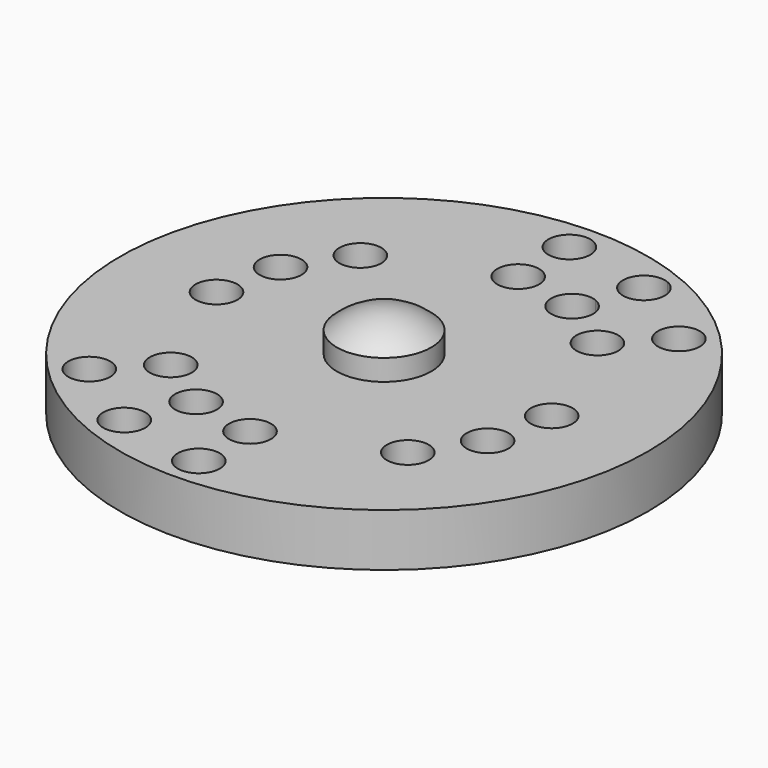
from build123d import *

# Parameters (mm, degrees)
F0_W     = 1.7891867319
F0_H     = 0.8
F2_R     = 0.79375
F3_DEPTH = 25.4


with BuildPart() as f1:
    # F0 (on Front) → F1 (revolve)
    with BuildSketch(Plane.XZ):
        with Locations((0.894593366, 0.4)):
            Rectangle(F0_W, F0_H)
        Polygon((1.7891867319, 0), (0, 0), (0, -3), (2.2, -3), (2.2, -2), (10, -2), (10, 0), align=None)
    revolve(axis=Axis((0, 0, -1.5), (0, 0, 1)))

    # F2 (on face) → F3 (cut)
    with BuildSketch(Plane.XY):
        with BuildLine():
            ThreePointArc((0.79375, 6.35), (-0.5612660076, 6.9112660076), (0, 5.55625))
            ThreePointArc((0, 5.55625), (0.5612660076, 5.7887339924), (0.79375, 6.35))
        make_face()
        with BuildLine():
            Line((2.4300397955, 5.8666350314), (2.1262848211, 5.1333056525))
            ThreePointArc((2.1262848211, 5.1333056525), (2.871023668, 5.2066560267), (3.2237897955, 5.8666350314))
            ThreePointArc((3.2237897955, 5.8666350314), (3.0900188003, 6.3076189039), (2.73379477, 6.5999644104))
            Line((2.73379477, 6.5999644104), (2.4300397955, 5.8666350314))
        make_face()
        with BuildLine():
            ThreePointArc((2.73379477, 6.5999644104), (1.6967104166, 6.1703900059), (2.1262848211, 5.1333056525))
            Line((2.1262848211, 5.1333056525), (2.4300397955, 5.8666350314))
            Line((2.4300397955, 5.8666350314), (2.73379477, 6.5999644104))
        make_face()
        with BuildLine():
            Line((4.4901280605, 4.4901280605), (3.928862053, 3.928862053))
            ThreePointArc((3.928862053, 3.928862053), (4.793883035, 3.7567986816), (5.2838780605, 4.4901280605))
            ThreePointArc((5.2838780605, 4.4901280605), (5.2234574395, 4.793883035), (5.0513940681, 5.0513940681))
            Line((5.0513940681, 5.0513940681), (4.4901280605, 4.4901280605))
        make_face()
        with BuildLine():
            ThreePointArc((5.0513940681, 5.0513940681), (3.928862053, 5.0513940681), (3.928862053, 3.928862053))
            Line((3.928862053, 3.928862053), (4.4901280605, 4.4901280605))
            Line((4.4901280605, 4.4901280605), (5.0513940681, 5.0513940681))
        make_face()
        with BuildLine():
            ThreePointArc((3.6618567991, 8.8405043479), (2.6247724457, 8.4109299434), (3.0543468502, 7.37384559))
            Line((3.0543468502, 7.37384559), (3.6618567991, 8.8405043479))
        make_face()
        with BuildLine():
            Line((3.6618567991, 8.8405043479), (3.0543468502, 7.37384559))
            ThreePointArc((3.0543468502, 7.37384559), (3.7990856971, 7.4471959642), (4.1518518247, 8.107174969))
            ThreePointArc((4.1518518247, 8.107174969), (4.0180808294, 8.5481588414), (3.6618567991, 8.8405043479))
        make_face()
        with BuildLine():
            ThreePointArc((6.7662290954, 6.7662290954), (5.6436970802, 6.7662290954), (5.6436970802, 5.6436970802))
            Line((5.6436970802, 5.6436970802), (6.7662290954, 6.7662290954))
        make_face()
        with BuildLine():
            Line((6.7662290954, 6.7662290954), (5.6436970802, 5.6436970802))
            ThreePointArc((5.6436970802, 5.6436970802), (6.5087180622, 5.4716337089), (6.9987130878, 6.2049630878))
            ThreePointArc((6.9987130878, 6.2049630878), (6.9382924667, 6.5087180622), (6.7662290954, 6.7662290954))
        make_face()
        with Locations((-6.35, 0)):
            Circle(F2_R)
        with Locations((-5.8666350314, 2.4300397955)):
            Circle(F2_R)
        with Locations((-4.4901280605, 4.4901280605)):
            Circle(F2_R)
        with Locations((0, -6.35)):
            Circle(F2_R)
        with Locations((-2.4300397955, -5.8666350314)):
            Circle(F2_R)
        with Locations((-4.4901280605, -4.4901280605)):
            Circle(F2_R)
        with Locations((6.35, 0)):
            Circle(F2_R)
        with Locations((5.8666350314, -2.4300397955)):
            Circle(F2_R)
        with Locations((4.4901280605, -4.4901280605)):
            Circle(F2_R)
        with Locations((0, 8.7751429528)):
            Circle(F2_R)
        with Locations((0, -8.7751429528)):
            Circle(F2_R)
        with Locations((-3.3581018247, -8.107174969)):
            Circle(F2_R)
        with Locations((-6.2049630878, -6.2049630878)):
            Circle(F2_R)
    extrude(amount=-F3_DEPTH, mode=Mode.SUBTRACT)

    # F4 (on Front) → F5 (revolve)
    with BuildSketch(Plane.XZ):
        with BuildLine():
            Line((-1.7891867319, 0.8), (0, 0.8))
            Line((0, 0.8), (0, 1.5092346721))
            ThreePointArc((0, 1.5092346721), (-0.9623153046, 1.3254595112), (-1.7891867319, 0.8))
        make_face()
    revolve(axis=Axis((0, 0, 1.1546173361), (0, 0, 1)))


solid = f1.part
